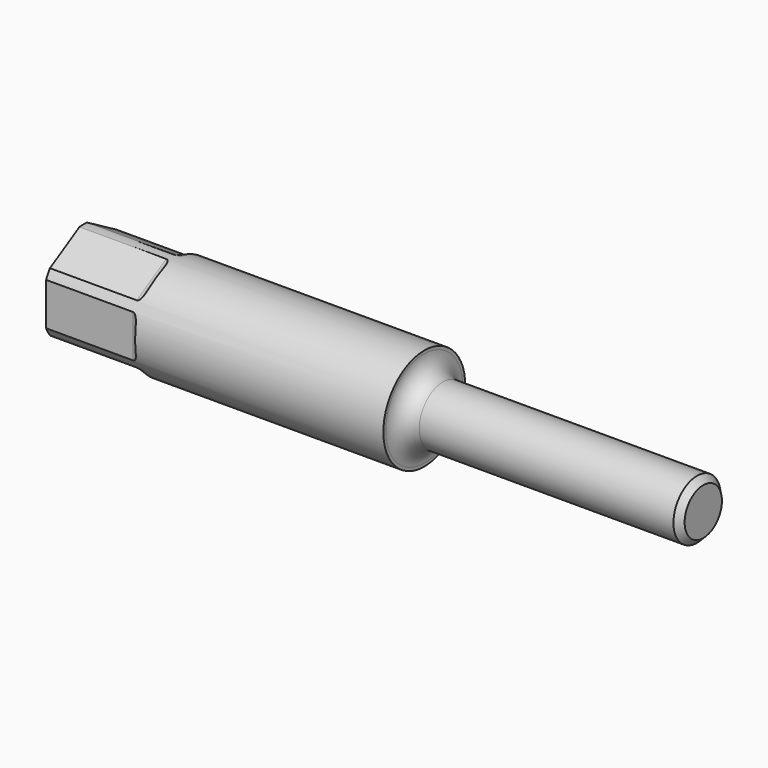
from build123d import *

# Parameters (mm, degrees)
F3_D         = 8.4328
F3_DEPTH     = 45
F3_TIP       = 2.5334687141
F2_R         = 25
F4_DEPTH     = 15
F5_T4_DEPTH  = 11.8738635424
F5_S5_R      = 8.25
F5_T6_DEPTH  = 8
F5_T10_DEPTH = 11.8738635424
F5_S11_R     = 8.25
F5_T12_DEPTH = 7
F5_T16_DEPTH = 11.8738635424
F5_S17_R     = 8.25
F5_T18_DEPTH = 8
F5_T22_DEPTH = 11.8738635424
F5_S23_R     = 8.25
F5_T24_DEPTH = 7
F5_T28_DEPTH = 11.8738635424
F5_S29_R     = 8.25
F5_T30_DEPTH = 8
F5_T34_DEPTH = 11.8738635424
F5_S35_R     = 8.25
F5_T36_DEPTH = 8
F6_SIZE      = 1
F7_R         = 3


# Not quite as in the source:
# - a fillet or chamfer that OpenCascade refuses, or shapes differently, is made with other operations: its cross-section is extruded or revolved along the edge and cut away or added


with BuildPart() as f1:
    # F0 (on Front) → F1 (revolve)
    with BuildSketch(Plane.XZ):
        Polygon((30, 8.25), (30, 0), (130, 0), (130, 4.7625), (85, 4.7625), (85, 8.25), align=None)
    revolve(axis=Axis((80, 0, 0), (-1, 0, 0)))

    # F3
    with Locations(Plane(origin=(30, 0, 0), x_dir=(0, -1, 0), z_dir=(-1, 0, 0))):
        with Locations((0, 0)):
            Hole(F3_D / 2, depth=F3_DEPTH)
            with Locations((0, 0, -(F3_DEPTH + F3_TIP / 2))):  # 118° drill point
                Cone(0, F3_D / 2, F3_TIP, mode=Mode.SUBTRACT)

    # F2 (on face) → F4 (cut)
    with BuildSketch(Plane(origin=(30, 0, 0), x_dir=(0, -1, 0), z_dir=(-1, 0, 0))):
        Circle(F2_R)
        with BuildLine():
            Line((6.7264702249, 4.7767246428), (7.5, 4.3301270189))
            Line((7.5, 4.3301270189), (7.5, 3.4369317712))
            ThreePointArc((7.5, 3.4369317712), (8.0603194726, 1.7589059099), (8.25, 0))
            ThreePointArc((8.25, 0), (8.0603194726, -1.7589059099), (7.5, -3.4369317712))
            Line((7.5, -3.4369317712), (7.5, -4.3301270189))
            Line((7.5, -4.3301270189), (6.7264702249, -4.7767246428))
            ThreePointArc((6.7264702249, -4.7767246428), (4.125, -7.1447095812), (0.7735297751, -8.213656414))
            Line((0.7735297751, -8.213656414), (0, -8.6602540378))
            Line((0, -8.6602540378), (-0.7735297751, -8.213656414))
            ThreePointArc((-0.7735297751, -8.213656414), (-4.125, -7.1447095812), (-6.7264702249, -4.7767246428))
            Line((-6.7264702249, -4.7767246428), (-7.5, -4.3301270189))
            Line((-7.5, -4.3301270189), (-7.5, -3.4369317712))
            ThreePointArc((-7.5, -3.4369317712), (-8.25, 0), (-7.5, 3.4369317712))
            Line((-7.5, 3.4369317712), (-7.5, 4.3301270189))
            Line((-7.5, 4.3301270189), (-6.7264702249, 4.7767246428))
            ThreePointArc((-6.7264702249, 4.7767246428), (-4.125, 7.1447095812), (-0.7735297751, 8.213656414))
            Line((-0.7735297751, 8.213656414), (0, 8.6602540378))
            Line((0, 8.6602540378), (0.7735297751, 8.213656414))
            ThreePointArc((0.7735297751, 8.213656414), (4.125, 7.1447095812), (6.7264702249, 4.7767246428))
        make_face(mode=Mode.SUBTRACT)
        with BuildLine():
            ThreePointArc((8.25, 0), (8.0603194726, 1.7589059099), (7.5, 3.4369317712))
            Line((7.5, 3.4369317712), (7.5, -3.4369317712))
            ThreePointArc((7.5, -3.4369317712), (8.0603194726, -1.7589059099), (8.25, 0))
        make_face()
        with BuildLine():
            Line((0.7735297751, 8.213656414), (6.7264702249, 4.7767246428))
            ThreePointArc((6.7264702249, 4.7767246428), (4.125, 7.1447095812), (0.7735297751, 8.213656414))
        make_face()
        with BuildLine():
            ThreePointArc((0.7735297751, -8.213656414), (4.125, -7.1447095812), (6.7264702249, -4.7767246428))
            Line((6.7264702249, -4.7767246428), (0.7735297751, -8.213656414))
        make_face()
        with BuildLine():
            Line((-6.7264702249, 4.7767246428), (-0.7735297751, 8.213656414))
            ThreePointArc((-0.7735297751, 8.213656414), (-4.125, 7.1447095812), (-6.7264702249, 4.7767246428))
        make_face()
        with BuildLine():
            ThreePointArc((-6.7264702249, -4.7767246428), (-4.125, -7.1447095812), (-0.7735297751, -8.213656414))
            Line((-0.7735297751, -8.213656414), (-6.7264702249, -4.7767246428))
        make_face()
        with BuildLine():
            Line((-7.5, -3.4369317712), (-7.5, 3.4369317712))
            ThreePointArc((-7.5, 3.4369317712), (-8.25, 0), (-7.5, -3.4369317712))
        make_face()
    extrude(amount=-F4_DEPTH, mode=Mode.SUBTRACT)

    # F5: fillet of radius 1 on 6 edges, made by hand


with BuildPart() as f5_tool2:
    # F5_s3 → F5_t4 (new body)
    with BuildSketch(Plane(origin=(0, 5.1415337344, 2.9684658856), x_dir=(1, 0, 0), z_dir=(0, -0.8660254038, -0.5))):
        with BuildLine():
            ThreePointArc((44, 7.5), (44.7071067812, 7.7928932188), (45, 8.5))
            Line((45, 8.5), (45, 7.5))
            Line((45, 7.5), (44, 7.5))
        make_face()
    extrude(amount=F5_T4_DEPTH)

    # F5_s5 → F5_t6 (intersect, symmetric)
    with BuildSketch(Plane.YZ.offset(44.5)):
        Circle(F5_S5_R)
    extrude(amount=F5_T6_DEPTH, both=True, mode=Mode.INTERSECT)


with BuildPart() as f1_1:
    add(f1.part)

    # F5_t1: union F5_tool2
    add(f5_tool2.part)


with BuildPart() as f5_tool8:
    # F5_s9 → F5_t10 (new body)
    with BuildSketch(Plane.XY.offset(5.9369317712)):
        with BuildLine():
            ThreePointArc((44, -7.5), (44.7071067812, -7.7928932188), (45, -8.5))
            Line((45, -8.5), (45, -7.5))
            Line((45, -7.5), (44, -7.5))
        make_face()
    extrude(amount=-F5_T10_DEPTH)

    # F5_s11 → F5_t12 (intersect, symmetric)
    with BuildSketch(Plane.YZ.offset(44.5)):
        Circle(F5_S11_R)
    extrude(amount=F5_T12_DEPTH, both=True, mode=Mode.INTERSECT)


with BuildPart() as f1_2:
    add(f1_1.part)

    # F5_t7: union F5_tool8
    add(f5_tool8.part)


with BuildPart() as f5_tool14:
    # F5_s15 → F5_t16 (new body)
    with BuildSketch(Plane(origin=(0, 5.1415337344, -2.9684658856), x_dir=(1, 0, 0), z_dir=(0, -0.8660254038, 0.5))):
        with BuildLine():
            ThreePointArc((44, 7.5), (44.7071067812, 7.7928932188), (45, 8.5))
            Line((45, 8.5), (45, 7.5))
            Line((45, 7.5), (44, 7.5))
        make_face()
    extrude(amount=F5_T16_DEPTH)

    # F5_s17 → F5_t18 (intersect, symmetric)
    with BuildSketch(Plane.YZ.offset(44.5)):
        Circle(F5_S17_R)
    extrude(amount=F5_T18_DEPTH, both=True, mode=Mode.INTERSECT)


with BuildPart() as f1_3:
    add(f1_2.part)

    # F5_t13: union F5_tool14
    add(f5_tool14.part)


with BuildPart() as f5_tool20:
    # F5_s21 → F5_t22 (new body)
    with BuildSketch(Plane.XY.offset(-5.9369317712)):
        with BuildLine():
            ThreePointArc((44, 7.5), (44.7071067812, 7.7928932188), (45, 8.5))
            Line((45, 8.5), (45, 7.5))
            Line((45, 7.5), (44, 7.5))
        make_face()
    extrude(amount=F5_T22_DEPTH)

    # F5_s23 → F5_t24 (intersect, symmetric)
    with BuildSketch(Plane.YZ.offset(44.5)):
        Circle(F5_S23_R)
    extrude(amount=F5_T24_DEPTH, both=True, mode=Mode.INTERSECT)


with BuildPart() as f1_4:
    add(f1_3.part)

    # F5_t19: union F5_tool20
    add(f5_tool20.part)


with BuildPart() as f5_tool26:
    # F5_s27 → F5_t28 (new body)
    with BuildSketch(Plane(origin=(0, -5.1415337344, -2.9684658856), x_dir=(1, 0, 0), z_dir=(0, 0.8660254038, 0.5))):
        with BuildLine():
            ThreePointArc((44, 7.5), (44.7071067812, 7.7928932188), (45, 8.5))
            Line((45, 8.5), (45, 7.5))
            Line((45, 7.5), (44, 7.5))
        make_face()
    extrude(amount=F5_T28_DEPTH)

    # F5_s29 → F5_t30 (intersect, symmetric)
    with BuildSketch(Plane.YZ.offset(44.5)):
        Circle(F5_S29_R)
    extrude(amount=F5_T30_DEPTH, both=True, mode=Mode.INTERSECT)


with BuildPart() as f1_5:
    add(f1_4.part)

    # F5_t25: union F5_tool26
    add(f5_tool26.part)


with BuildPart() as f5_tool32:
    # F5_s33 → F5_t34 (new body)
    with BuildSketch(Plane(origin=(0, -5.1415337344, 2.9684658856), x_dir=(1, 0, 0), z_dir=(0, 0.8660254038, -0.5))):
        with BuildLine():
            ThreePointArc((44, 7.5), (44.7071067812, 7.7928932188), (45, 8.5))
            Line((45, 8.5), (45, 7.5))
            Line((45, 7.5), (44, 7.5))
        make_face()
    extrude(amount=F5_T34_DEPTH)

    # F5_s35 → F5_t36 (intersect, symmetric)
    with BuildSketch(Plane.YZ.offset(44.5)):
        Circle(F5_S35_R)
    extrude(amount=F5_T36_DEPTH, both=True, mode=Mode.INTERSECT)


with BuildPart() as f1_6:
    add(f1_5.part)

    # F5_t31: union F5_tool32
    add(f5_tool32.part)

    # F6
    f6_edges = [f1_6.edges().sort_by_distance(p)[0] for p in [
        (130, 0, -4.7625),
    ]]
    chamfer(f6_edges, length=F6_SIZE)

    # F7
    f7_edges = [f1_6.edges().sort_by_distance(p)[0] for p in [
        (85, 0, -4.7625),
    ]]
    fillet(f7_edges, radius=F7_R)


solid = f1_6.part
